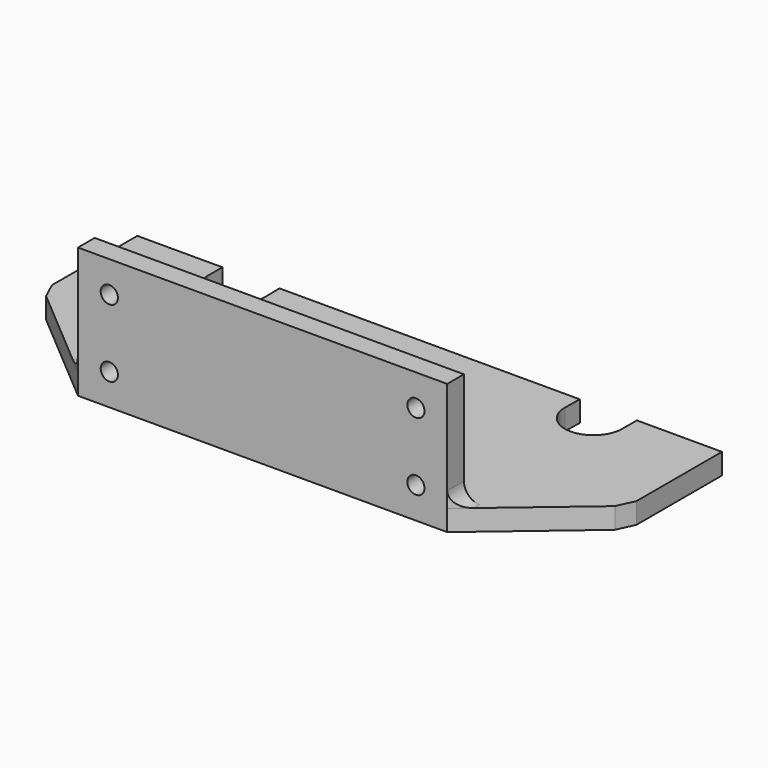
from build123d import *

# Parameters (mm, degrees)
F0_R     = 2.5
F0_R_2   = 2
F1_DEPTH = 4
F3_DEPTH = 21
F5_DEPTH = 25
F6_D     = 3.3
F7_SIZE  = 2


# Not quite as in the source:
# - ends of sketch curves that miss each other by under 0.0002 mm in the source are joined


with BuildPart() as f1:
    # F0 (on Top) → F1 (new body)
    with BuildSketch(Plane.XY):
        with BuildLine():
            ThreePointArc((0, 18.5), (13.081475452, 13.081475452), (18.5, 0))
            ThreePointArc((18.5, 0), (-1.1345020789, -18.4651808828), (-18.3608545982, 2.2647336323))
            ThreePointArc((-18.3608545982, 2.2647336323), (-20.315445832, 5.8895882396), (-20.061448931, 9.9999998237))
            ThreePointArc((-20.061448931, 9.9999998237), (-38.4593739655, 0.6163893281), (-48.7895366382, 18.5))
            Line((-48.7895366382, 18.5), (-55, 18.5))
            Line((-55, 18.5), (-55, -3.5))
            Line((-55, -3.5), (-35, -20.5))
            Line((-35, -20.5), (0, -20.5))
            Line((0, -20.5), (35, -20.5))
            Line((35, -20.5), (55, -3.5))
            Line((55, -3.5), (55, 18.5))
            Line((55, 18.5), (39.703517094, 18.5))
            Line((39.703517094, 18.5), (39.703517094, 15))
            ThreePointArc((39.703517094, 15), (39.7035676427, 14.9863858353), (39.703517094, 14.9727717541))
            ThreePointArc((39.703517094, 14.9727717541), (34.1416723213, 9.5003484762), (28.7044327696, 15.096593634))
            Line((28.7044327696, 15.096593634), (28.7642142424, 18.5))
            Line((28.7642142424, 18.5), (0, 18.5))
        make_face()
        with BuildLine():
            ThreePointArc((-18.3608545982, 2.2647336323), (-1.1345020789, -18.4651808828), (18.5, 0))
            ThreePointArc((18.5, 0), (13.081475452, 13.081475452), (0, 18.5))
            ThreePointArc((0, 18.5), (-5.8749853417, 17.542364357), (-11.1417441574, 14.7685997011))
            ThreePointArc((-11.1417441574, 14.7685997011), (-7.0694530575, 12.1035433774), (-5.4903810568, 7.5))
            ThreePointArc((-5.4903810568, 7.5), (-5.7459373553, 5.5588571779), (-6.4951905116, 3.750000029))
            ThreePointArc((-6.4951905116, 3.750000029), (-12.0588494406, 0.0580749232), (-18.3608545982, 2.2647336323))
        make_face()
        with BuildLine():
            ThreePointArc((7.5, 0), (-1.9411428544, -7.2444436928), (-6.4951905116, 3.750000029))
            ThreePointArc((-6.4951905116, 3.750000029), (1.9411428544, 7.2444436928), (7.5, 0))
        make_face(mode=Mode.SUBTRACT)
        with BuildLine():
            ThreePointArc((7.5, 0), (1.9411428544, 7.2444436928), (-6.4951905116, 3.750000029))
            ThreePointArc((-6.4951905116, 3.750000029), (-1.9411428544, -7.2444436928), (7.5, 0))
        make_face()
        Circle(F0_R, mode=Mode.SUBTRACT)
        with BuildLine():
            ThreePointArc((-11.1417441574, 14.7685997011), (-16.02146997, 9.25), (-18.3608545982, 2.2647336323))
            ThreePointArc((-18.3608545982, 2.2647336323), (-12.0588494406, 0.0580749232), (-6.4951905116, 3.750000029))
            ThreePointArc((-6.4951905116, 3.750000029), (-5.7459373553, 5.5588571779), (-5.4903810568, 7.5))
            ThreePointArc((-5.4903810568, 7.5), (-7.0694530575, 12.1035433774), (-11.1417441574, 14.7685997011))
        make_face()
        with Locations((-12.9903810568, 7.5)):
            Circle(F0_R_2, mode=Mode.SUBTRACT)
        with BuildLine():
            ThreePointArc((-20.061448931, 9.9999998237), (-20.315445832, 5.8895882396), (-18.3608545982, 2.2647336323))
            ThreePointArc((-18.3608545982, 2.2647336323), (-16.02146997, 9.25), (-11.1417441574, 14.7685997011))
            ThreePointArc((-11.1417441574, 14.7685997011), (-16.5263862207, 14.1141263581), (-20.061448931, 9.9999998237))
        make_face()
        with BuildLine():
            ThreePointArc((-11.1417441574, 14.7685997011), (-5.8749853417, 17.542364357), (0, 18.5))
            Line((0, 18.5), (-19.6176323465, 18.5))
            ThreePointArc((-19.6176323465, 18.5), (-19.3074560996, 16.7622028562), (-19.2035844924, 15))
            ThreePointArc((-19.2035844924, 15), (-19.4196061134, 12.463470227), (-20.061448931, 9.9999998237))
            ThreePointArc((-20.061448931, 9.9999998237), (-16.5263862207, 14.1141263581), (-11.1417441574, 14.7685997011))
        make_face()
        with BuildLine():
            ThreePointArc((-19.2035844924, 15), (-19.3074560996, 16.7622028562), (-19.6176323465, 18.5))
            Line((-19.6176323465, 18.5), (-28.7642142424, 18.5))
            Line((-28.7642142424, 18.5), (-28.7044327696, 15.096593634))
            ThreePointArc((-28.7044327696, 15.096593634), (-28.7037965658, 15.0482986794), (-28.7035844924, 15))
            ThreePointArc((-28.7035844924, 15), (-34.1899703277, 9.5000168496), (-39.703517094, 14.9727717541))
            Line((-39.703517094, 14.9727717541), (-39.703517094, 18.5))
            Line((-39.703517094, 18.5), (-48.7895366382, 18.5))
            ThreePointArc((-48.7895366382, 18.5), (-38.4593739655, 0.6163893281), (-20.061448931, 9.9999998237))
            ThreePointArc((-20.061448931, 9.9999998237), (-19.4196061134, 12.463470227), (-19.2035844924, 15))
        make_face()
        Polygon((-55, -3.5), (-55, 18.5), (-56, 18.5), (-56, -3.9624404748), (-35.3675770292, -21.5), (0, -21.5), (35.3675770292, -21.5), (56, -3.9624404748), (56, 18.5), (55, 18.5), (55, -3.5), (35, -20.5), (0, -20.5), (-35, -20.5), align=None)
    extrude(amount=F1_DEPTH)

    # F2 (on face) → F3 (join)
    with BuildSketch(Plane.XY.offset(4)):
        Polygon((40.0734593822, -17.5), (-40.0734593822, -17.5), (-35.3675770292, -21.5), (35.3675770292, -21.5), align=None)
    extrude(amount=F3_DEPTH)

    # F4 (on face) → F5 (cut)
    with BuildSketch(Plane.XZ.offset(21.5)):
        with BuildLine():
            Line((-35.3675770292, 25), (-40.0734593822, 25))
            Line((-40.0734593822, 25), (-40.0734593822, 4))
            Line((-40.0734593822, 4), (-38.3675770292, 4))
            ThreePointArc((-38.3675770292, 4), (-36.2462566857, 4.8786796564), (-35.3675770292, 7))
            Line((-35.3675770292, 7), (-35.3675770292, 25))
        make_face()
        with BuildLine():
            Line((40.0734593822, 25), (35.3675770292, 25))
            Line((35.3675770292, 25), (35.3675770292, 7))
            ThreePointArc((35.3675770292, 7), (36.2462566857, 4.8786796564), (38.3675770292, 4))
            Line((38.3675770292, 4), (40.0734593822, 4))
            Line((40.0734593822, 4), (40.0734593822, 25))
        make_face()
    extrude(amount=-F5_DEPTH, mode=Mode.SUBTRACT)

    # F6 (through all)
    with Locations(Plane.XZ.offset(21.5)):
        with Locations((-29.3675770292, 19), (-29.3675770292, 6), (29.3675770292, 6), (29.3675770292, 19)):
            Hole(F6_D / 2)

    # F7
    f7_edges = [f1.edges().sort_by_distance(p)[0] for p in [
        (-56, -3.96244, 2),
        (56, -3.96244, 2),
    ]]
    chamfer(f7_edges, length=F7_SIZE)


solid = f1.part
